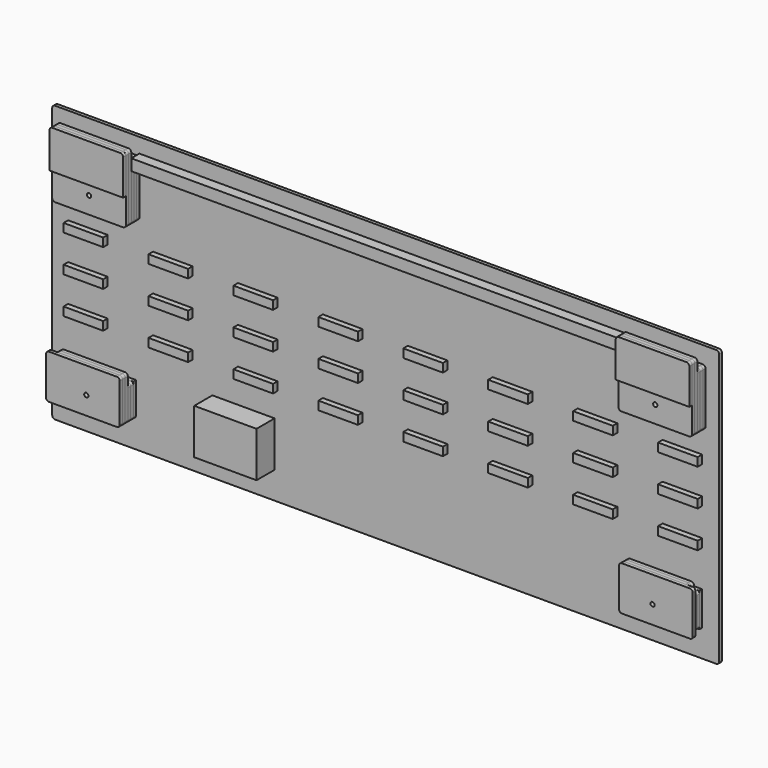
from build123d import *

# Parameters (mm, degrees)
F0_W      = 1178
F0_H      = 488
F1_DEPTH  = 6
F2_W      = 70
F2_H      = 15
F3_DEPTH  = 10
F4_W      = 130
F4_H      = 100
F5_DEPTH  = 6
F4_W_2    = 118
F4_H_2    = 60
F6_DEPTH  = 6
F7_R      = 5
F7_2_R    = 5
F8_W      = 130
F8_H      = 100
F9_DEPTH  = 6
F8_W_2    = 118
F8_H_2    = 60
F10_W     = 130
F10_H     = 100
F11_DEPTH = 6
F10_W_2   = 118
F10_H_2   = 60
F12_W     = 130
F12_H     = 118
F13_DEPTH = 6
F12_W_2   = 118
F12_H_2   = 78
F14_W     = 130
F14_H     = 118
F15_DEPTH = 6
F14_W_2   = 118
F14_H_2   = 78
F16_R     = 5
F16_2_R   = 5
F16_3_R   = 5
F16_4_R   = 5
F16_5_R   = 5
F16_6_R   = 5
F16_7_R   = 5
F16_8_R   = 5
F16_9_R   = 5
F16_10_R  = 5
F16_11_R  = 5
F16_12_R  = 5
F16_13_R  = 5
F16_14_R  = 5
F16_15_R  = 5
F17_R     = 5
F17_2_R   = 5
F17_3_R   = 5
F17_4_R   = 5
F17_5_R   = 5
F18_W     = 129.9603307247
F18_H     = 118
F19_DEPTH = 6
F18_W_2   = 130.0539374352
F18_H_2   = 78.0870169401
F20_R     = 5
F20_2_R   = 5
F21_R     = 5
F21_2_R   = 5
F22_R     = 3.75
F23_DEPTH = 50
F24_W     = 110
F24_H     = 80
F25_DEPTH = 40
F26_R     = 5
F27_W     = 870.0793385506
F27_H     = 20
F28_DEPTH = 18
F30_R     = 5
F31_W     = 129.9603307247
F31_H     = 50
F32_DEPTH = 6


# Not quite as in the source:
# - a feature names something its author has since deleted; it is built from what else it names
# - the program builds the solid bodies; features that only make, move or delete a surface that nothing else refers to are left out


with BuildPart() as f1:
    # F0 (on Front) → F1 (new body)
    with BuildSketch(Plane.XZ):
        Rectangle(F0_W, F0_H)
    extrude(amount=F1_DEPTH)


with BuildPart() as f3:
    # F2 (on face) → F3 (new body)
    with BuildSketch(Plane.XZ.offset(6)):
        with Locations((-526.0000860691, 65.8508732915)):
            Rectangle(F2_W, F2_H)
    extrude(amount=F3_DEPTH)


with BuildPart() as f3b:
    # F2 (on face) → F3, piece 2 (new body)
    with BuildSketch(Plane.XZ.offset(6)):
        with Locations((-526.0000860691, 0.8508732915)):
            Rectangle(F2_W, F2_H)
    extrude(amount=F3_DEPTH)


with BuildPart() as f3c:
    # F2 (on face) → F3, piece 3 (new body)
    with BuildSketch(Plane.XZ.offset(6)):
        with Locations((-526.0000860691, -64.1491267085)):
            Rectangle(F2_W, F2_H)
    extrude(amount=F3_DEPTH)


with BuildPart() as f3d:
    # F2 (on face) → F3, piece 4 (new body)
    with BuildSketch(Plane.XZ.offset(6)):
        with Locations((-376.0000860691, 65.8508732915)):
            Rectangle(F2_W, F2_H)
    extrude(amount=F3_DEPTH)


with BuildPart() as f3e:
    # F2 (on face) → F3, piece 5 (new body)
    with BuildSketch(Plane.XZ.offset(6)):
        with Locations((-376.0000860691, 0.8508732915)):
            Rectangle(F2_W, F2_H)
    extrude(amount=F3_DEPTH)


with BuildPart() as f3f:
    # F2 (on face) → F3, piece 6 (new body)
    with BuildSketch(Plane.XZ.offset(6)):
        with Locations((-376.0000860691, -64.1491267085)):
            Rectangle(F2_W, F2_H)
    extrude(amount=F3_DEPTH)


with BuildPart() as f3g:
    # F2 (on face) → F3, piece 7 (new body)
    with BuildSketch(Plane.XZ.offset(6)):
        with Locations((-226.0000860691, 65.8508732915)):
            Rectangle(F2_W, F2_H)
    extrude(amount=F3_DEPTH)


with BuildPart() as f3h:
    # F2 (on face) → F3, piece 8 (new body)
    with BuildSketch(Plane.XZ.offset(6)):
        with Locations((-226.0000860691, 0.8508732915)):
            Rectangle(F2_W, F2_H)
    extrude(amount=F3_DEPTH)


with BuildPart() as f3i:
    # F2 (on face) → F3, piece 9 (new body)
    with BuildSketch(Plane.XZ.offset(6)):
        with Locations((-226.0000860691, -64.1491267085)):
            Rectangle(F2_W, F2_H)
    extrude(amount=F3_DEPTH)


with BuildPart() as f3j:
    # F2 (on face) → F3, piece 10 (new body)
    with BuildSketch(Plane.XZ.offset(6)):
        with Locations((-76.0000860691, 65.8508732915)):
            Rectangle(F2_W, F2_H)
    extrude(amount=F3_DEPTH)


with BuildPart() as f3k:
    # F2 (on face) → F3, piece 11 (new body)
    with BuildSketch(Plane.XZ.offset(6)):
        with Locations((-76.0000860691, 0.8508732915)):
            Rectangle(F2_W, F2_H)
    extrude(amount=F3_DEPTH)


with BuildPart() as f3l:
    # F2 (on face) → F3, piece 12 (new body)
    with BuildSketch(Plane.XZ.offset(6)):
        with Locations((-76.0000860691, -64.1491267085)):
            Rectangle(F2_W, F2_H)
    extrude(amount=F3_DEPTH)


with BuildPart() as f3m:
    # F2 (on face) → F3, piece 13 (new body)
    with BuildSketch(Plane.XZ.offset(6)):
        with Locations((73.9999139309, 65.8508732915)):
            Rectangle(F2_W, F2_H)
    extrude(amount=F3_DEPTH)


with BuildPart() as f3n:
    # F2 (on face) → F3, piece 14 (new body)
    with BuildSketch(Plane.XZ.offset(6)):
        with Locations((73.9999139309, 0.8508732915)):
            Rectangle(F2_W, F2_H)
    extrude(amount=F3_DEPTH)


with BuildPart() as f3o:
    # F2 (on face) → F3, piece 15 (new body)
    with BuildSketch(Plane.XZ.offset(6)):
        with Locations((73.9999139309, -64.1491267085)):
            Rectangle(F2_W, F2_H)
    extrude(amount=F3_DEPTH)


with BuildPart() as f3p:
    # F2 (on face) → F3, piece 16 (new body)
    with BuildSketch(Plane.XZ.offset(6)):
        with Locations((223.9999139309, 65.8508732915)):
            Rectangle(F2_W, F2_H)
    extrude(amount=F3_DEPTH)


with BuildPart() as f3q:
    # F2 (on face) → F3, piece 17 (new body)
    with BuildSketch(Plane.XZ.offset(6)):
        with Locations((223.9999139309, 0.8508732915)):
            Rectangle(F2_W, F2_H)
    extrude(amount=F3_DEPTH)


with BuildPart() as f3r:
    # F2 (on face) → F3, piece 18 (new body)
    with BuildSketch(Plane.XZ.offset(6)):
        with Locations((223.9999139309, -64.1491267085)):
            Rectangle(F2_W, F2_H)
    extrude(amount=F3_DEPTH)


with BuildPart() as f3s:
    # F2 (on face) → F3, piece 19 (new body)
    with BuildSketch(Plane.XZ.offset(6)):
        with Locations((373.9999139309, 65.8508732915)):
            Rectangle(F2_W, F2_H)
    extrude(amount=F3_DEPTH)


with BuildPart() as f3t:
    # F2 (on face) → F3, piece 20 (new body)
    with BuildSketch(Plane.XZ.offset(6)):
        with Locations((373.9999139309, 0.8508732915)):
            Rectangle(F2_W, F2_H)
    extrude(amount=F3_DEPTH)


with BuildPart() as f3u:
    # F2 (on face) → F3, piece 21 (new body)
    with BuildSketch(Plane.XZ.offset(6)):
        with Locations((373.9999139309, -64.1491267085)):
            Rectangle(F2_W, F2_H)
    extrude(amount=F3_DEPTH)


with BuildPart() as f3v:
    # F2 (on face) → F3, piece 22 (new body)
    with BuildSketch(Plane.XZ.offset(6)):
        with Locations((523.9999139309, 65.8508732915)):
            Rectangle(F2_W, F2_H)
    extrude(amount=F3_DEPTH)


with BuildPart() as f3w:
    # F2 (on face) → F3, piece 23 (new body)
    with BuildSketch(Plane.XZ.offset(6)):
        with Locations((523.9999139309, 0.8508732915)):
            Rectangle(F2_W, F2_H)
    extrude(amount=F3_DEPTH)


with BuildPart() as f3x:
    # F2 (on face) → F3, piece 24 (new body)
    with BuildSketch(Plane.XZ.offset(6)):
        with Locations((523.9999139309, -64.1491267085)):
            Rectangle(F2_W, F2_H)
    extrude(amount=F3_DEPTH)


with BuildPart() as f5:
    # F4 (on face) → F5 (new body)
    with BuildSketch(Plane.XZ.offset(6)):
        with Locations((-500, 164)):
            Rectangle(F4_W, F4_H)
    extrude(amount=F5_DEPTH)

    # F7
    f7_edges = [f5.edges().sort_by_distance(p)[0] for p in [
        (-565, -9, 214),
        (-565, -9, 114),
        (-435, -9, 214),
        (-435, -9, 114),
    ]]
    fillet(f7_edges, radius=F7_R)


with BuildPart() as f5b:
    # F4 (on face) → F5, piece 2 (new body)
    with BuildSketch(Plane.XZ.offset(6)):
        with Locations((500, 164)):
            Rectangle(F4_W, F4_H)
    extrude(amount=F5_DEPTH)

    # F7#2
    f7_2_edges = [f5b.edges().sort_by_distance(p)[0] for p in [
        (435, -9, 114),
        (565, -9, 114),
        (435, -9, 214),
        (565, -9, 214),
    ]]
    fillet(f7_2_edges, radius=F7_2_R)


with BuildPart() as f5c:
    # F4 (on face) → F5, piece 3 (new body)
    with BuildSketch(Plane.XZ.offset(6)):
        with Locations((-500, -166)):
            Rectangle(F4_W_2, F4_H_2)
    extrude(amount=F5_DEPTH)

    # F16#6
    f16_6_edges = [f5c.edges().sort_by_distance(p)[0] for p in [
        (-559, -9, -136),
        (-559, -9, -196),
        (-441, -9, -196),
        (-441, -9, -136),
    ]]
    fillet(f16_6_edges, radius=F16_6_R)


with BuildPart() as f5d:
    # F4 (on face) → F5, piece 4 (new body)
    with BuildSketch(Plane.XZ.offset(6)):
        with Locations((500, -166)):
            Rectangle(F4_W_2, F4_H_2)
    extrude(amount=F5_DEPTH)

    # F16#15
    f16_15_edges = [f5d.edges().sort_by_distance(p)[0] for p in [
        (559, -9, -136),
        (559, -9, -196),
        (441, -9, -196),
        (441, -9, -136),
    ]]
    fillet(f16_15_edges, radius=F16_15_R)


with BuildPart() as f6:
    # F4 (on face) → F6 (new body)
    with BuildSketch(Plane.XZ.offset(6)):
        with Locations((-500, 164)):
            Rectangle(F4_W, F4_H)
    extrude(amount=F6_DEPTH)

    # F16#5
    f16_5_edges = [f6.edges().sort_by_distance(p)[0] for p in [
        (-435, -9, 114),
    ]]
    fillet(f16_5_edges, radius=F16_5_R)


with BuildPart() as f6b:
    # F4 (on face) → F6, piece 2 (new body)
    with BuildSketch(Plane.XZ.offset(6)):
        with Locations((500, 164)):
            Rectangle(F4_W, F4_H)
    extrude(amount=F6_DEPTH)

    # F17#5
    f17_5_edges = [f6b.edges().sort_by_distance(p)[0] for p in [
        (565, -9, 114),
        (565, -9, 214),
        (435, -9, 214),
        (435, -9, 114),
    ]]
    fillet(f17_5_edges, radius=F17_5_R)


with BuildPart() as f6c:
    # F4 (on face) → F6, piece 3 (new body)
    with BuildSketch(Plane.XZ.offset(6)):
        with Locations((-500, -166)):
            Rectangle(F4_W_2, F4_H_2)
    extrude(amount=F6_DEPTH)


with BuildPart() as f6d:
    # F4 (on face) → F6, piece 4 (new body)
    with BuildSketch(Plane.XZ.offset(6)):
        with Locations((500, -166)):
            Rectangle(F4_W_2, F4_H_2)
    extrude(amount=F6_DEPTH)


with BuildPart() as f9:
    # F8 (on face) → F9 (new body)
    with BuildSketch(Plane.XZ.offset(12)):
        with Locations((-500, 164)):
            Rectangle(F8_W, F8_H)
    extrude(amount=F9_DEPTH)

    # F16
    f16_edges = [f9.edges().sort_by_distance(p)[0] for p in [
        (-565, -15, 214),
        (-565, -15, 114),
        (-435, -15, 114),
        (-435, -15, 214),
    ]]
    fillet(f16_edges, radius=F16_R)


with BuildPart() as f9b:
    # F8 (on face) → F9, piece 2 (new body)
    with BuildSketch(Plane.XZ.offset(12)):
        with Locations((500, 164)):
            Rectangle(F8_W, F8_H)
    extrude(amount=F9_DEPTH)

    # F17
    f17_edges = [f9b.edges().sort_by_distance(p)[0] for p in [
        (565, -15, 114),
        (565, -15, 214),
        (435, -15, 214),
        (435, -15, 114),
    ]]
    fillet(f17_edges, radius=F17_R)


with BuildPart() as f9c:
    # F8 (on face) → F9, piece 3 (new body)
    with BuildSketch(Plane.XZ.offset(12)):
        with Locations((-500, -166)):
            Rectangle(F8_W_2, F8_H_2)
    extrude(amount=F9_DEPTH)

    # F16#7
    f16_7_edges = [f9c.edges().sort_by_distance(p)[0] for p in [
        (-559, -15, -136),
        (-559, -15, -196),
        (-441, -15, -196),
        (-441, -15, -136),
    ]]
    fillet(f16_7_edges, radius=F16_7_R)


with BuildPart() as f9d:
    # F8 (on face) → F9, piece 4 (new body)
    with BuildSketch(Plane.XZ.offset(12)):
        with Locations((500, -166)):
            Rectangle(F8_W_2, F8_H_2)
    extrude(amount=F9_DEPTH)

    # F16#14
    f16_14_edges = [f9d.edges().sort_by_distance(p)[0] for p in [
        (559, -15, -136),
        (559, -15, -196),
        (441, -15, -196),
        (441, -15, -136),
    ]]
    fillet(f16_14_edges, radius=F16_14_R)


with BuildPart() as f11:
    # F10 (on face) → F11 (new body)
    with BuildSketch(Plane.XZ.offset(18)):
        with Locations((-500, 164)):
            Rectangle(F10_W, F10_H)
    extrude(amount=F11_DEPTH)

    # F16#2
    f16_2_edges = [f11.edges().sort_by_distance(p)[0] for p in [
        (-565, -21, 214),
        (-565, -21, 114),
        (-435, -21, 114),
        (-435, -21, 214),
    ]]
    fillet(f16_2_edges, radius=F16_2_R)


with BuildPart() as f11b:
    # F10 (on face) → F11, piece 2 (new body)
    with BuildSketch(Plane.XZ.offset(18)):
        with Locations((500, 164)):
            Rectangle(F10_W, F10_H)
    extrude(amount=F11_DEPTH)

    # F17#2
    f17_2_edges = [f11b.edges().sort_by_distance(p)[0] for p in [
        (565, -21, 114),
        (565, -21, 214),
        (435, -21, 214),
        (435, -21, 114),
    ]]
    fillet(f17_2_edges, radius=F17_2_R)


with BuildPart() as f11c:
    # F10 (on face) → F11, piece 3 (new body)
    with BuildSketch(Plane.XZ.offset(18)):
        with Locations((-500, -166)):
            Rectangle(F10_W_2, F10_H_2)
    extrude(amount=F11_DEPTH)

    # F16#8
    f16_8_edges = [f11c.edges().sort_by_distance(p)[0] for p in [
        (-559, -21, -136),
        (-559, -21, -196),
        (-441, -21, -196),
        (-441, -21, -136),
    ]]
    fillet(f16_8_edges, radius=F16_8_R)


with BuildPart() as f11d:
    # F10 (on face) → F11, piece 4 (new body)
    with BuildSketch(Plane.XZ.offset(18)):
        with Locations((500, -166)):
            Rectangle(F10_W_2, F10_H_2)
    extrude(amount=F11_DEPTH)

    # F16#13
    f16_13_edges = [f11d.edges().sort_by_distance(p)[0] for p in [
        (559, -21, -136),
        (559, -21, -196),
        (441, -21, -196),
        (441, -21, -136),
    ]]
    fillet(f16_13_edges, radius=F16_13_R)


with BuildPart() as f13:
    # F12 (on face) → F13 (new body)
    with BuildSketch(Plane.XZ.offset(24)):
        with Locations((-500, 173)):
            Rectangle(F12_W, F12_H)
    extrude(amount=F13_DEPTH)

    # F16#3
    f16_3_edges = [f13.edges().sort_by_distance(p)[0] for p in [
        (-565, -27, 232),
        (-565, -27, 114),
        (-435, -27, 114),
        (-435, -27, 232),
    ]]
    fillet(f16_3_edges, radius=F16_3_R)


with BuildPart() as f13b:
    # F12 (on face) → F13, piece 2 (new body)
    with BuildSketch(Plane.XZ.offset(24)):
        with Locations((500, 173)):
            Rectangle(F12_W, F12_H)
    extrude(amount=F13_DEPTH)

    # F17#3
    f17_3_edges = [f13b.edges().sort_by_distance(p)[0] for p in [
        (565, -27, 114),
        (565, -27, 232),
        (435, -27, 232),
        (435, -27, 114),
    ]]
    fillet(f17_3_edges, radius=F17_3_R)


with BuildPart() as f13c:
    # F12 (on face) → F13, piece 3 (new body)
    with BuildSketch(Plane.XZ.offset(24)):
        with Locations((-500, -157)):
            Rectangle(F12_W_2, F12_H_2)
    extrude(amount=F13_DEPTH)

    # F16#9
    f16_9_edges = [f13c.edges().sort_by_distance(p)[0] for p in [
        (-559, -27, -118),
        (-559, -27, -196),
        (-441, -27, -196),
        (-441, -27, -118),
    ]]
    fillet(f16_9_edges, radius=F16_9_R)


with BuildPart() as f13d:
    # F12 (on face) → F13, piece 4 (new body)
    with BuildSketch(Plane.XZ.offset(24)):
        with Locations((500, -157)):
            Rectangle(F12_W_2, F12_H_2)
    extrude(amount=F13_DEPTH)

    # F16#12
    f16_12_edges = [f13d.edges().sort_by_distance(p)[0] for p in [
        (559, -27, -118),
        (559, -27, -196),
        (441, -27, -196),
        (441, -27, -118),
    ]]
    fillet(f16_12_edges, radius=F16_12_R)


with BuildPart() as f15:
    # F14 (on face) → F15 (new body)
    with BuildSketch(Plane.XZ.offset(30)):
        with Locations((-500, 173)):
            Rectangle(F14_W, F14_H)
    extrude(amount=F15_DEPTH)

    # F16#4
    f16_4_edges = [f15.edges().sort_by_distance(p)[0] for p in [
        (-565, -33, 232),
        (-565, -33, 114),
        (-435, -33, 114),
        (-435, -33, 232),
    ]]
    fillet(f16_4_edges, radius=F16_4_R)


with BuildPart() as f15b:
    # F14 (on face) → F15, piece 2 (new body)
    with BuildSketch(Plane.XZ.offset(30)):
        with Locations((500, 173)):
            Rectangle(F14_W, F14_H)
    extrude(amount=F15_DEPTH)

    # F17#4
    f17_4_edges = [f15b.edges().sort_by_distance(p)[0] for p in [
        (565, -33, 114),
        (565, -33, 232),
        (435, -33, 232),
        (435, -33, 114),
    ]]
    fillet(f17_4_edges, radius=F17_4_R)


with BuildPart() as f15c:
    # F14 (on face) → F15, piece 3 (new body)
    with BuildSketch(Plane.XZ.offset(30)):
        with Locations((-500, -157)):
            Rectangle(F14_W_2, F14_H_2)
    extrude(amount=F15_DEPTH)

    # F16#10
    f16_10_edges = [f15c.edges().sort_by_distance(p)[0] for p in [
        (-559, -33, -118),
        (-559, -33, -196),
        (-441, -33, -196),
        (-441, -33, -118),
    ]]
    fillet(f16_10_edges, radius=F16_10_R)


with BuildPart() as f15d:
    # F14 (on face) → F15, piece 4 (new body)
    with BuildSketch(Plane.XZ.offset(30)):
        with Locations((500, -157)):
            Rectangle(F14_W_2, F14_H_2)
    extrude(amount=F15_DEPTH)

    # F16#11
    f16_11_edges = [f15d.edges().sort_by_distance(p)[0] for p in [
        (559, -33, -118),
        (559, -33, -196),
        (441, -33, -196),
        (441, -33, -118),
    ]]
    fillet(f16_11_edges, radius=F16_11_R)


with BuildPart() as f19:
    # F18 (on face) → F19 (new body)
    with BuildSketch(Plane.XZ.offset(36)):
        with Locations((-500.0198346376, 173)):
            Rectangle(F18_W, F18_H)
    extrude(amount=F19_DEPTH)

    # F20
    f20_edges = [f19.edges().sort_by_distance(p)[0] for p in [
        (-435.039669, -39, 232),
        (-565, -39, 232),
        (-565, -39, 114),
        (-435.039669, -39, 114),
    ]]
    fillet(f20_edges, radius=F20_R)


with BuildPart() as f19b:
    # F18 (on face) → F19, piece 2 (new body)
    with BuildSketch(Plane.XZ.offset(36)):
        with Locations((500.0198346376, 173)):
            Rectangle(F18_W, F18_H)
    extrude(amount=F19_DEPTH)

    # F20#2
    f20_2_edges = [f19b.edges().sort_by_distance(p)[0] for p in [
        (565, -39, 114),
        (435.039669, -39, 114),
        (435.039669, -39, 232),
        (565, -39, 232),
    ]]
    fillet(f20_2_edges, radius=F20_2_R)


with BuildPart() as f19c:
    # F18 (on face) → F19, piece 3 (new body)
    with BuildSketch(Plane.XZ.offset(36)):
        with Locations((-506.0269687176, -156.9564915299)):
            Rectangle(F18_W_2, F18_H_2)
    extrude(amount=F19_DEPTH)

    # F21
    f21_edges = [f19c.edges().sort_by_distance(p)[0] for p in [
        (-441, -39, -117.912983),
        (-441, -39, -196),
        (-571.053937, -39, -117.912983),
        (-571.053937, -39, -196),
    ]]
    fillet(f21_edges, radius=F21_R)


with BuildPart() as f19d:
    # F18 (on face) → F19, piece 4 (new body)
    with BuildSketch(Plane.XZ.offset(36)):
        with Locations((506.0269687176, -156.9564915299)):
            Rectangle(F18_W_2, F18_H_2)
    extrude(amount=F19_DEPTH)

    # F21#2
    f21_2_edges = [f19d.edges().sort_by_distance(p)[0] for p in [
        (441, -39, -117.912983),
        (441, -39, -196),
        (571.053937, -39, -196),
        (571.053937, -39, -117.912983),
    ]]
    fillet(f21_2_edges, radius=F21_2_R)


with BuildPart() as f23_tool:
    # F22 (on face) → F23 (new body)
    with BuildSketch(Plane.XZ.offset(42)):
        with Locations((-500, 144)):
            Circle(F22_R)
        with Locations((500, 144)):
            Circle(F22_R)
        with Locations((-500, -164)):
            Circle(F22_R)
        with Locations((500, -164)):
            Circle(F22_R)
    extrude(amount=-F23_DEPTH)


with BuildPart() as f1_1:
    add(f1.part)

    # F23: cut by f23_tool
    add(f23_tool.part, mode=Mode.SUBTRACT)

    # F30
    f30_edges = [f1_1.edges().sort_by_distance(p)[0] for p in [
        (-589, -3, 244),
        (-589, -3, -244),
        (589, -3, 244),
        (589, -3, -244),
    ]]
    fillet(f30_edges, radius=F30_R)


with BuildPart() as f5_1:
    add(f5.part)

    # F23: cut by f23_tool
    add(f23_tool.part, mode=Mode.SUBTRACT)


with BuildPart() as f5b_1:
    add(f5b.part)

    # F23: cut by f23_tool
    add(f23_tool.part, mode=Mode.SUBTRACT)


with BuildPart() as f5c_1:
    add(f5c.part)

    # F23: cut by f23_tool
    add(f23_tool.part, mode=Mode.SUBTRACT)


with BuildPart() as f5d_1:
    add(f5d.part)

    # F23: cut by f23_tool
    add(f23_tool.part, mode=Mode.SUBTRACT)


with BuildPart() as f6_1:
    add(f6.part)

    # F23: cut by f23_tool
    add(f23_tool.part, mode=Mode.SUBTRACT)


with BuildPart() as f6b_1:
    add(f6b.part)

    # F23: cut by f23_tool
    add(f23_tool.part, mode=Mode.SUBTRACT)


with BuildPart() as f6c_1:
    add(f6c.part)

    # F23: cut by f23_tool
    add(f23_tool.part, mode=Mode.SUBTRACT)

    # F26
    f26_edges = [f6c_1.edges().sort_by_distance(p)[0] for p in [
        (-441, -9, -196),
    ]]
    fillet(f26_edges, radius=F26_R)


with BuildPart() as f6d_1:
    add(f6d.part)

    # F23: cut by f23_tool
    add(f23_tool.part, mode=Mode.SUBTRACT)


with BuildPart() as f9_1:
    add(f9.part)

    # F23: cut by f23_tool
    add(f23_tool.part, mode=Mode.SUBTRACT)


with BuildPart() as f9b_1:
    add(f9b.part)

    # F23: cut by f23_tool
    add(f23_tool.part, mode=Mode.SUBTRACT)


with BuildPart() as f9c_1:
    add(f9c.part)

    # F23: cut by f23_tool
    add(f23_tool.part, mode=Mode.SUBTRACT)


with BuildPart() as f9d_1:
    add(f9d.part)

    # F23: cut by f23_tool
    add(f23_tool.part, mode=Mode.SUBTRACT)


with BuildPart() as f11_1:
    add(f11.part)

    # F23: cut by f23_tool
    add(f23_tool.part, mode=Mode.SUBTRACT)


with BuildPart() as f11b_1:
    add(f11b.part)

    # F23: cut by f23_tool
    add(f23_tool.part, mode=Mode.SUBTRACT)


with BuildPart() as f11c_1:
    add(f11c.part)

    # F23: cut by f23_tool
    add(f23_tool.part, mode=Mode.SUBTRACT)


with BuildPart() as f11d_1:
    add(f11d.part)

    # F23: cut by f23_tool
    add(f23_tool.part, mode=Mode.SUBTRACT)


with BuildPart() as f13_1:
    add(f13.part)

    # F23: cut by f23_tool
    add(f23_tool.part, mode=Mode.SUBTRACT)


with BuildPart() as f13b_1:
    add(f13b.part)

    # F23: cut by f23_tool
    add(f23_tool.part, mode=Mode.SUBTRACT)


with BuildPart() as f13c_1:
    add(f13c.part)

    # F23: cut by f23_tool
    add(f23_tool.part, mode=Mode.SUBTRACT)


with BuildPart() as f13d_1:
    add(f13d.part)

    # F23: cut by f23_tool
    add(f23_tool.part, mode=Mode.SUBTRACT)


with BuildPart() as f15_1:
    add(f15.part)

    # F23: cut by f23_tool
    add(f23_tool.part, mode=Mode.SUBTRACT)


with BuildPart() as f15b_1:
    add(f15b.part)

    # F23: cut by f23_tool
    add(f23_tool.part, mode=Mode.SUBTRACT)


with BuildPart() as f15c_1:
    add(f15c.part)

    # F23: cut by f23_tool
    add(f23_tool.part, mode=Mode.SUBTRACT)


with BuildPart() as f15d_1:
    add(f15d.part)

    # F23: cut by f23_tool
    add(f23_tool.part, mode=Mode.SUBTRACT)


with BuildPart() as f19_1:
    add(f19.part)

    # F23: cut by f23_tool
    add(f23_tool.part, mode=Mode.SUBTRACT)


with BuildPart() as f19b_1:
    add(f19b.part)

    # F23: cut by f23_tool
    add(f23_tool.part, mode=Mode.SUBTRACT)


with BuildPart() as f19c_1:
    add(f19c.part)

    # F23: cut by f23_tool
    add(f23_tool.part, mode=Mode.SUBTRACT)


with BuildPart() as f19d_1:
    add(f19d.part)

    # F23: cut by f23_tool
    add(f23_tool.part, mode=Mode.SUBTRACT)


with BuildPart() as f25:
    # F24 (on face) → F25 (new body)
    with BuildSketch(Plane.XZ.offset(6)):
        with Locations((-251.1978596449, -156)):
            Rectangle(F24_W, F24_H)
    extrude(amount=F25_DEPTH)


with BuildPart() as f28:
    # F27 (on face) → F28 (new body)
    with BuildSketch(Plane.XZ.offset(6)):
        with Locations((0, 208)):
            Rectangle(F27_W, F27_H)
    extrude(amount=F28_DEPTH)


with BuildPart() as f32_tool:
    # F31 (on face) → F32 (new body)
    with BuildSketch(Plane.XZ.offset(42)):
        with Locations((-500.0198346376, 139)):
            Rectangle(F31_W, F31_H)
        with Locations((500.0198346376, 139)):
            Rectangle(F31_W, F31_H)
    extrude(amount=-F32_DEPTH)


with BuildPart() as f19_2:
    add(f19_1.part)

    # F32: cut by f32_tool
    add(f32_tool.part, mode=Mode.SUBTRACT)


with BuildPart() as f19b_2:
    add(f19b_1.part)

    # F32: cut by f32_tool
    add(f32_tool.part, mode=Mode.SUBTRACT)


solid = Compound([f3.part, f3b.part, f3c.part, f3d.part, f3e.part, f3f.part, f3g.part, f3h.part, f3i.part, f3j.part, f3k.part, f3l.part, f3m.part, f3n.part, f3o.part, f3p.part, f3q.part, f3r.part, f3s.part, f3t.part, f3u.part, f3v.part, f3w.part, f3x.part, f1_1.part, f5_1.part, f5b_1.part, f5c_1.part, f5d_1.part, f6_1.part, f6b_1.part, f6c_1.part, f6d_1.part, f9_1.part, f9b_1.part, f9c_1.part, f9d_1.part, f11_1.part, f11b_1.part, f11c_1.part, f11d_1.part, f13_1.part, f13b_1.part, f13c_1.part, f13d_1.part, f15_1.part, f15b_1.part, f15c_1.part, f15d_1.part, f19c_1.part, f19d_1.part, f25.part, f28.part, f19_2.part, f19b_2.part])
